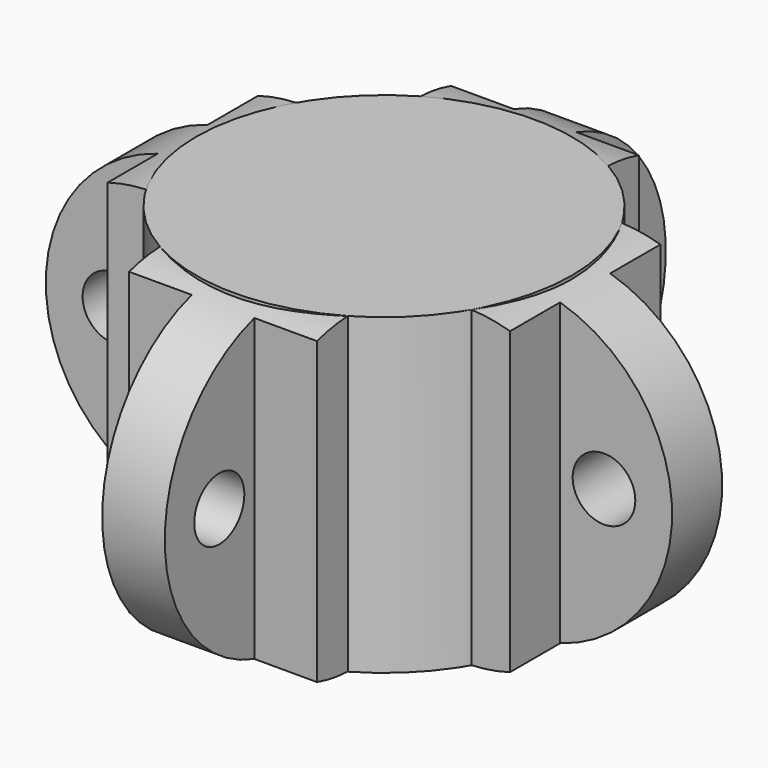
from build123d import *

# Parameters (mm, degrees)
F0_W            = 25
F0_H            = 50
F0_R            = 5
F1_DEPTH        = 15
F1_DEPTH_BACK   = 15
F2_COUNT        = 2
F2_ANGLE        = 90
F3_R            = 30
F4_DEPTH        = 50
F5_W            = 36.1747656763
F5_H            = 34.8211117089
F5_W_2          = 32.0865538716
F5_H_2          = 43.4180013835
F6_DEPTH        = 50.0010001
F6_COPIES_COUNT = 4


# Not quite as in the source:
# - a pattern or mirror of a feature is missing from the dataset's text; its kind, count and spacing are read off the source's solid


with BuildPart() as f1:
    # F0 (on Front) → F1 (new body, two sides)
    with BuildSketch(Plane.XZ) as f1_sk:
        with Locations((-12.5, 25)):
            Rectangle(F0_W, F0_H)
        with Locations((12.5, 25)):
            Rectangle(F0_W, F0_H)
        with BuildLine():
            ThreePointArc((-25, 50), (-50, 25), (-25, 0))
            Line((-25, 0), (-25, 50))
        make_face()
        with Locations((-39.1249991953, 25)):
            Circle(F0_R, mode=Mode.SUBTRACT)
        with BuildLine():
            Line((25, 50), (25, 0))
            ThreePointArc((25, 0), (50, 25), (25, 50))
        make_face()
        with Locations((39.1249991953, 25)):
            Circle(F0_R, mode=Mode.SUBTRACT)
    extrude(amount=F1_DEPTH)
    extrude(f1_sk.sketch, amount=-F1_DEPTH_BACK)

    # F2: F1 ×2 about axis
    f2_axis = Axis((0, 0, 10.6249991804), (0, 0, 1))


with BuildPart() as f1_1:
    add(f1.part)
    for i in range(1, F2_COUNT):
        add(f1.part.rotate(f2_axis, i * F2_ANGLE / (F2_COUNT - 1)))

    # F3 (on face) → F4 (join, through all)
    with BuildSketch(Plane.XY.offset(50)):
        Circle(F3_R)
    extrude(amount=-F4_DEPTH)

    # F5 (on face) → F6 (cut, through all)
    with BuildSketch(Plane.XY.offset(50)):
        with Locations((-23.0873828381, 49.535555765)):
            Rectangle(F5_W, F5_H)
        with Locations((21.0432769358, 53.8340006024)):
            Rectangle(F5_W_2, F5_H_2)
    f6 = extrude(amount=-F6_DEPTH, mode=Mode.SUBTRACT)

    # F6_copies: F6 ×4 about axis
    f6_copies_axis = Axis((0, 0, 0), (0, 0, 1))
    for i in range(1, F6_COPIES_COUNT):
        add(f6.rotate(f6_copies_axis, i * 360 / F6_COPIES_COUNT), mode=Mode.SUBTRACT)


solid = f1_1.part
